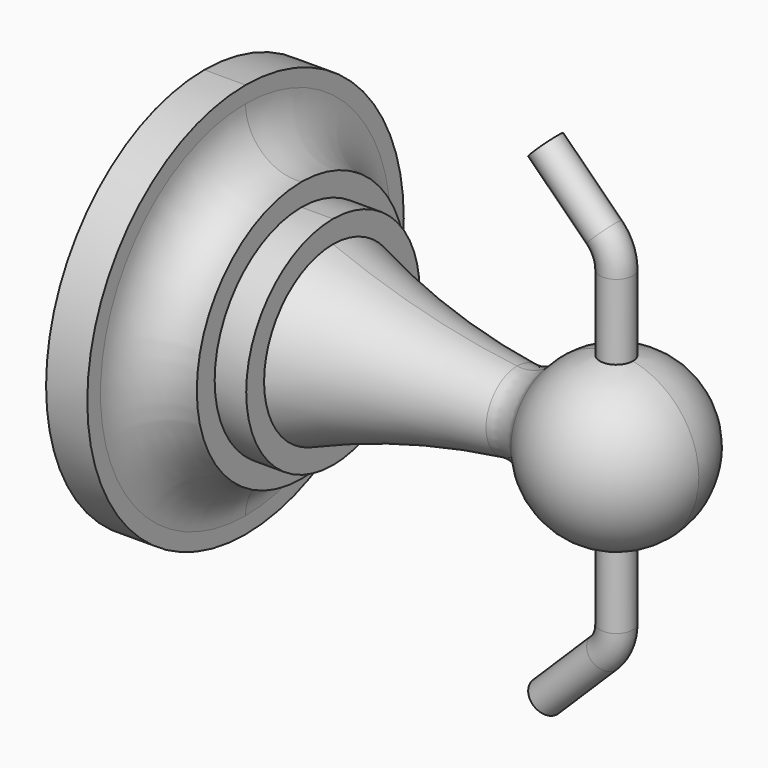
from build123d import *
from build123d import SkipClean  # not in build123d's __all__

# Parameters (mm, degrees)
F2_R          = 5
F3_R          = 2
F4_DEPTH      = 25
F4_DEPTH_BACK = 25
F6_R          = 2


with BuildPart() as f1:
    # F0 (on Front) → F1 (revolve)
    with BuildSketch(Plane.XZ):
        with BuildLine():
            Line((-60, 0), (0, 0))
            ThreePointArc((0, 0), (-7.7499262393, 9.7435706018), (-18.9874336143, 4.3847505093))
            ThreePointArc((-18.9874336143, 4.3847505093), (-31.9220569404, 6.4479089357), (-44.3965084851, 10.4415491223))
            Line((-44.3965084851, 10.4415491223), (-44.3965084851, 13.1515692919))
            Line((-44.3965084851, 13.1515692919), (-48.2224225998, 13.1515692919))
            Line((-48.2224225998, 13.1515692919), (-48.2224225998, 15.8615894616))
            ThreePointArc((-48.2224225998, 15.8615894616), (-52.9723552194, 17.427920622), (-55, 22))
            Line((-55, 22), (-55, 24))
            Line((-55, 24), (-60, 24))
            Line((-60, 24), (-60, 0))
        make_face()
    revolve(axis=Axis((-30, 0, 0), (-1, 0, 0)))

    # F2
    f2_edges = [f1.edges().sort_by_distance(p)[0] for p in [
        (-18.987434, 0, -4.384751),
    ]]
    fillet(f2_edges, radius=F2_R)

    # F3 (on Top) → F4 (cut, two sides)
    with BuildSketch(Plane.XY) as f4_sk:
        with Locations((-10, 0)):
            Circle(F3_R)
    extrude(amount=-F4_DEPTH, mode=Mode.SUBTRACT)
    extrude(f4_sk.sketch, amount=F4_DEPTH_BACK, mode=Mode.SUBTRACT)

    # F7: sweep along a path in F5
    with BuildLine(Plane.XZ) as f7_path:
        Line((-10, 0), (-10, -18.9135132155))
        ThreePointArc((-10, -18.9135132155), (-10.3850895053, -20.8377276333), (-11.4810404502, -22.4655441398))
        Line((-11.4810404502, -22.4655441398), (-18.572177738, -29.4906590134))
    # F6 (on Top) → F7 (sweep)
    with BuildSketch(Plane.XY):
        with Locations((-10, 0)):
            Circle(F6_R)
    sweep(path=f7_path.line)

    # F8: F1 across plane


with BuildPart() as f1_1:
    add(f1.part, clean=False)
    with SkipClean():  # cleaning this boolean's faces spoils the solid; the shape is the same uncleaned
        add(f1.part.mirror(Plane.XY), clean=False)


solid = f1_1.part
